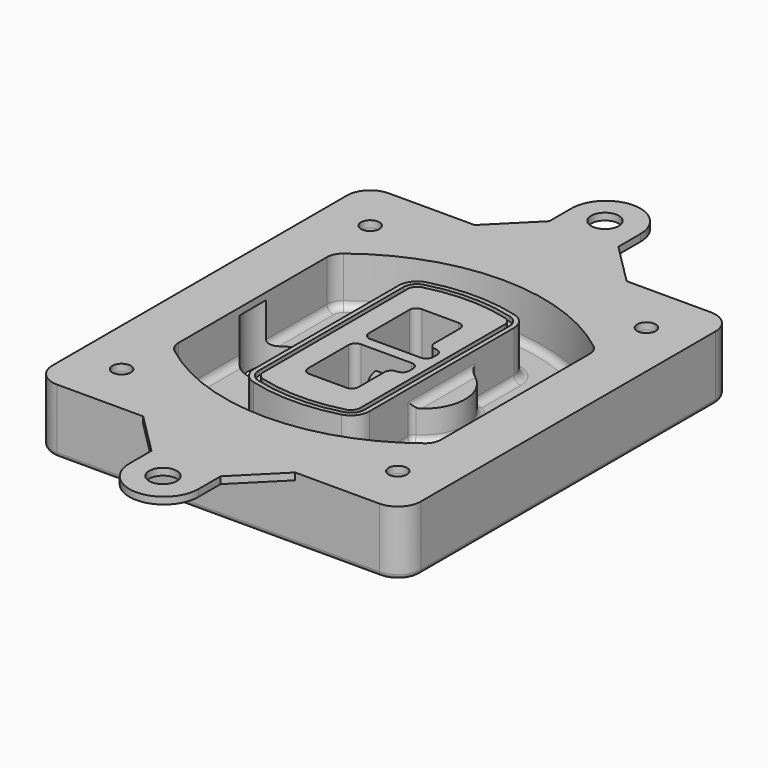
from build123d import *

# Parameters (mm, degrees)
F0_R      = 4
F1_DEPTH  = 25
F2_DEPTH  = 3
F3_DEPTH  = 18
F5_DEPTH  = 21
F6_DEPTH  = 2
F8_DEPTH  = 20
F9_DEPTH  = 16
F10_DEPTH = 25
F7_R      = 6
F7_R_2    = 4
F11_DEPTH = 6
F13_DEPTH = 9
F14_R     = 2
F15_R     = 3
F16_R     = 4
F16_R_2   = 6.0213144339
F17_DEPTH = 3


# Not quite as in the source:
# - a feature names something its author has since deleted; it is built from what else it names


with BuildPart() as f1:
    # F0 (on Top) → F1 (new body)
    with BuildSketch(Plane.XY):
        with BuildLine():
            ThreePointArc((-80, -80), (-77.0710678119, -87.0710678119), (-70, -90))
            Line((-70, -90), (70, -90))
            ThreePointArc((70, -90), (77.0710678119, -87.0710678119), (80, -80))
            Line((80, -80), (80, 80))
            ThreePointArc((80, 80), (77.0710678119, 87.0710678119), (70, 90))
            Line((70, 90), (-70, 90))
            ThreePointArc((-70, 90), (-77.0710678119, 87.0710678119), (-80, 80))
            Line((-80, 80), (-80, -80))
        make_face()
        with Locations((-60, -67.5)):
            Circle(F0_R, mode=Mode.SUBTRACT)
        with Locations((60, -67.5)):
            Circle(F0_R, mode=Mode.SUBTRACT)
        with Locations((-60, 67.5)):
            Circle(F0_R, mode=Mode.SUBTRACT)
        with BuildLine():
            ThreePointArc((-64, 40.2934422872), (-62.5820384798, 46.4328484224), (-58.6153846154, 51.3286200352))
            ThreePointArc((-58.6153846154, 51.3286200352), (0, 71.5), (58.6153846154, 51.3286200352))
            ThreePointArc((58.6153846154, 51.3286200352), (62.5820384798, 46.4328484224), (64, 40.2934422872))
            Line((64, 40.2934422872), (64, -40.2934422872))
            ThreePointArc((64, -40.2934422872), (62.5820384798, -46.4328484224), (58.6153846154, -51.3286200352))
            ThreePointArc((58.6153846154, -51.3286200352), (0, -71.5), (-58.6153846154, -51.3286200352))
            ThreePointArc((-58.6153846154, -51.3286200352), (-62.5820384798, -46.4328484224), (-64, -40.2934422872))
            Line((-64, -40.2934422872), (-64, 40.2934422872))
        make_face(mode=Mode.SUBTRACT)
        with Locations((60, 67.5)):
            Circle(F0_R, mode=Mode.SUBTRACT)
        with BuildLine():
            ThreePointArc((58.6153846154, 51.3286200352), (0, 71.5), (-58.6153846154, 51.3286200352))
            ThreePointArc((-58.6153846154, 51.3286200352), (-62.5820384798, 46.4328484224), (-64, 40.2934422872))
            Line((-64, 40.2934422872), (-64, -40.2934422872))
            ThreePointArc((-64, -40.2934422872), (-62.5820384798, -46.4328484224), (-58.6153846154, -51.3286200352))
            ThreePointArc((-58.6153846154, -51.3286200352), (0, -71.5), (58.6153846154, -51.3286200352))
            ThreePointArc((58.6153846154, -51.3286200352), (62.5820384798, -46.4328484224), (64, -40.2934422872))
            Line((64, -40.2934422872), (64, 40.2934422872))
            ThreePointArc((64, 40.2934422872), (62.5820384798, 46.4328484224), (58.6153846154, 51.3286200352))
        make_face()
        with BuildLine():
            Line((-60, -40.2934422872), (-60, 40.2934422872))
            ThreePointArc((-60, 40.2934422872), (-58.9871703427, 44.6787323838), (-56.1538461538, 48.1757121072))
            ThreePointArc((-56.1538461538, 48.1757121072), (0, 67.5), (56.1538461538, 48.1757121072))
            ThreePointArc((56.1538461538, 48.1757121072), (58.9871703427, 44.6787323838), (60, 40.2934422872))
            Line((60, 40.2934422872), (60, -40.2934422872))
            ThreePointArc((60, -40.2934422872), (58.9871703427, -44.6787323838), (56.1538461538, -48.1757121072))
            ThreePointArc((56.1538461538, -48.1757121072), (0, -67.5), (-56.1538461538, -48.1757121072))
            ThreePointArc((-56.1538461538, -48.1757121072), (-58.9871703427, -44.6787323838), (-60, -40.2934422872))
        make_face(mode=Mode.SUBTRACT)
        with BuildLine():
            ThreePointArc((-56.1538461538, 48.1757121072), (-58.9871703427, 44.6787323838), (-60, 40.2934422872))
            Line((-60, 40.2934422872), (-60, -40.2934422872))
            ThreePointArc((-60, -40.2934422872), (-58.9871703427, -44.6787323838), (-56.1538461538, -48.1757121072))
            ThreePointArc((-56.1538461538, -48.1757121072), (0, -67.5), (56.1538461538, -48.1757121072))
            ThreePointArc((56.1538461538, -48.1757121072), (58.9871703427, -44.6787323838), (60, -40.2934422872))
            Line((60, -40.2934422872), (60, 40.2934422872))
            ThreePointArc((60, 40.2934422872), (58.9871703427, 44.6787323838), (56.1538461538, 48.1757121072))
            ThreePointArc((56.1538461538, 48.1757121072), (0, 67.5), (-56.1538461538, 48.1757121072))
        make_face()
        with BuildLine():
            ThreePointArc((54.3076923077, 45.8110311612), (56.2910192399, 43.3631453548), (57, 40.2934422872))
            Line((57, 40.2934422872), (57, -40.2934422872))
            ThreePointArc((57, -40.2934422872), (56.2910192399, -43.3631453548), (54.3076923077, -45.8110311612))
            ThreePointArc((54.3076923077, -45.8110311612), (0, -64.5), (-54.3076923077, -45.8110311612))
            ThreePointArc((-54.3076923077, -45.8110311612), (-56.2910192399, -43.3631453548), (-57, -40.2934422872))
            Line((-57, -40.2934422872), (-57, 40.2934422872))
            ThreePointArc((-57, 40.2934422872), (-56.2910192399, 43.3631453548), (-54.3076923077, 45.8110311612))
            ThreePointArc((-54.3076923077, 45.8110311612), (0, 64.5), (54.3076923077, 45.8110311612))
        make_face(mode=Mode.SUBTRACT)
        with BuildLine():
            Line((57, -40.2934422872), (57, 40.2934422872))
            ThreePointArc((57, 40.2934422872), (56.2910192399, 43.3631453548), (54.3076923077, 45.8110311612))
            ThreePointArc((54.3076923077, 45.8110311612), (0, 64.5), (-54.3076923077, 45.8110311612))
            ThreePointArc((-54.3076923077, 45.8110311612), (-56.2910192399, 43.3631453548), (-57, 40.2934422872))
            Line((-57, 40.2934422872), (-57, -40.2934422872))
            ThreePointArc((-57, -40.2934422872), (-56.2910192399, -43.3631453548), (-54.3076923077, -45.8110311612))
            ThreePointArc((-54.3076923077, -45.8110311612), (0, -64.5), (54.3076923077, -45.8110311612))
            ThreePointArc((54.3076923077, -45.8110311612), (56.2910192399, -43.3631453548), (57, -40.2934422872))
        make_face()
    extrude(amount=-F1_DEPTH)

    # F0 (on Top) → F2 (join)
    with BuildSketch(Plane.XY):
        with BuildLine():
            ThreePointArc((-56.1538461538, 48.1757121072), (-58.9871703427, 44.6787323838), (-60, 40.2934422872))
            Line((-60, 40.2934422872), (-60, -40.2934422872))
            ThreePointArc((-60, -40.2934422872), (-58.9871703427, -44.6787323838), (-56.1538461538, -48.1757121072))
            ThreePointArc((-56.1538461538, -48.1757121072), (0, -67.5), (56.1538461538, -48.1757121072))
            ThreePointArc((56.1538461538, -48.1757121072), (58.9871703427, -44.6787323838), (60, -40.2934422872))
            Line((60, -40.2934422872), (60, 40.2934422872))
            ThreePointArc((60, 40.2934422872), (58.9871703427, 44.6787323838), (56.1538461538, 48.1757121072))
            ThreePointArc((56.1538461538, 48.1757121072), (0, 67.5), (-56.1538461538, 48.1757121072))
        make_face()
        with BuildLine():
            ThreePointArc((54.3076923077, 45.8110311612), (56.2910192399, 43.3631453548), (57, 40.2934422872))
            Line((57, 40.2934422872), (57, -40.2934422872))
            ThreePointArc((57, -40.2934422872), (56.2910192399, -43.3631453548), (54.3076923077, -45.8110311612))
            ThreePointArc((54.3076923077, -45.8110311612), (0, -64.5), (-54.3076923077, -45.8110311612))
            ThreePointArc((-54.3076923077, -45.8110311612), (-56.2910192399, -43.3631453548), (-57, -40.2934422872))
            Line((-57, -40.2934422872), (-57, 40.2934422872))
            ThreePointArc((-57, 40.2934422872), (-56.2910192399, 43.3631453548), (-54.3076923077, 45.8110311612))
            ThreePointArc((-54.3076923077, 45.8110311612), (0, 64.5), (54.3076923077, 45.8110311612))
        make_face(mode=Mode.SUBTRACT)
    extrude(amount=F2_DEPTH)

    # F0 (on Top) → F3 (cut)
    with BuildSketch(Plane.XY):
        with BuildLine():
            Line((57, -40.2934422872), (57, 40.2934422872))
            ThreePointArc((57, 40.2934422872), (56.2910192399, 43.3631453548), (54.3076923077, 45.8110311612))
            ThreePointArc((54.3076923077, 45.8110311612), (0, 64.5), (-54.3076923077, 45.8110311612))
            ThreePointArc((-54.3076923077, 45.8110311612), (-56.2910192399, 43.3631453548), (-57, 40.2934422872))
            Line((-57, 40.2934422872), (-57, -40.2934422872))
            ThreePointArc((-57, -40.2934422872), (-56.2910192399, -43.3631453548), (-54.3076923077, -45.8110311612))
            ThreePointArc((-54.3076923077, -45.8110311612), (0, -64.5), (54.3076923077, -45.8110311612))
            ThreePointArc((54.3076923077, -45.8110311612), (56.2910192399, -43.3631453548), (57, -40.2934422872))
        make_face()
    extrude(amount=-F3_DEPTH, mode=Mode.SUBTRACT)

    # F4 (on face) → F5 (join, through all)
    with BuildSketch(Plane.XY.offset(3)):
        with BuildLine():
            ThreePointArc((-25, -39.2465276821), (-23.3511545998, -44.1109737193), (-19.0842911877, -46.9702398883))
            ThreePointArc((-19.0842911877, -46.9702398883), (0, -49.5), (19.0842911877, -46.9702398883))
            ThreePointArc((19.0842911877, -46.9702398883), (23.3511545998, -44.1109737193), (25, -39.2465276821))
            Line((25, -39.2465276821), (25, 39.2465276821))
            ThreePointArc((25, 39.2465276821), (23.3511545998, 44.1109737193), (19.0842911877, 46.9702398883))
            ThreePointArc((19.0842911877, 46.9702398883), (0, 49.5), (-19.0842911877, 46.9702398883))
            ThreePointArc((-19.0842911877, 46.9702398883), (-23.3511545998, 44.1109737193), (-25, 39.2465276821))
            Line((-25, 39.2465276821), (-25, -39.2465276821))
        make_face()
        with BuildLine():
            ThreePointArc((18.5632183908, 45.0393118368), (21.7633659499, 42.89486221), (23, 39.2465276821))
            Line((23, 39.2465276821), (23, -39.2465276821))
            ThreePointArc((23, -39.2465276821), (21.7633659499, -42.89486221), (18.5632183908, -45.0393118368))
            ThreePointArc((18.5632183908, -45.0393118368), (0, -47.5), (-18.5632183908, -45.0393118368))
            ThreePointArc((-18.5632183908, -45.0393118368), (-21.7633659499, -42.89486221), (-23, -39.2465276821))
            Line((-23, -39.2465276821), (-23, 39.2465276821))
            ThreePointArc((-23, 39.2465276821), (-21.7633659499, 42.89486221), (-18.5632183908, 45.0393118368))
            ThreePointArc((-18.5632183908, 45.0393118368), (0, 47.5), (18.5632183908, 45.0393118368))
        make_face(mode=Mode.SUBTRACT)
        with BuildLine():
            Line((23, -39.2465276821), (23, 39.2465276821))
            ThreePointArc((23, 39.2465276821), (21.7633659499, 42.89486221), (18.5632183908, 45.0393118368))
            ThreePointArc((18.5632183908, 45.0393118368), (0, 47.5), (-18.5632183908, 45.0393118368))
            ThreePointArc((-18.5632183908, 45.0393118368), (-21.7633659499, 42.89486221), (-23, 39.2465276821))
            Line((-23, 39.2465276821), (-23, -39.2465276821))
            ThreePointArc((-23, -39.2465276821), (-21.7633659499, -42.89486221), (-18.5632183908, -45.0393118368))
            ThreePointArc((-18.5632183908, -45.0393118368), (0, -47.5), (18.5632183908, -45.0393118368))
            ThreePointArc((18.5632183908, -45.0393118368), (21.7633659499, -42.89486221), (23, -39.2465276821))
        make_face()
        with BuildLine():
            ThreePointArc((18.0421455939, 43.1083837852), (20.1755772999, 41.6787507007), (21, 39.2465276821))
            Line((21, 39.2465276821), (21, -39.2465276821))
            ThreePointArc((21, -39.2465276821), (20.1755772999, -41.6787507007), (18.0421455939, -43.1083837852))
            ThreePointArc((18.0421455939, -43.1083837852), (0, -45.5), (-18.0421455939, -43.1083837852))
            ThreePointArc((-18.0421455939, -43.1083837852), (-20.1755772999, -41.6787507007), (-21, -39.2465276821))
            Line((-21, -39.2465276821), (-21, 39.2465276821))
            ThreePointArc((-21, 39.2465276821), (-20.1755772999, 41.6787507007), (-18.0421455939, 43.1083837852))
            ThreePointArc((-18.0421455939, 43.1083837852), (0, 45.5), (18.0421455939, 43.1083837852))
        make_face(mode=Mode.SUBTRACT)
        with BuildLine():
            Line((21, -39.2465276821), (21, 39.2465276821))
            ThreePointArc((21, 39.2465276821), (20.1755772999, 41.6787507007), (18.0421455939, 43.1083837852))
            ThreePointArc((18.0421455939, 43.1083837852), (0, 45.5), (-18.0421455939, 43.1083837852))
            ThreePointArc((-18.0421455939, 43.1083837852), (-20.1755772999, 41.6787507007), (-21, 39.2465276821))
            Line((-21, 39.2465276821), (-21, -39.2465276821))
            ThreePointArc((-21, -39.2465276821), (-20.1755772999, -41.6787507007), (-18.0421455939, -43.1083837852))
            ThreePointArc((-18.0421455939, -43.1083837852), (0, -45.5), (18.0421455939, -43.1083837852))
            ThreePointArc((18.0421455939, -43.1083837852), (20.1755772999, -41.6787507007), (21, -39.2465276821))
        make_face()
        with BuildLine():
            Line((-8, -2.5), (14, -2.5))
            ThreePointArc((14, -2.5), (16.1213203436, -3.3786796564), (17, -5.5))
            Line((17, -5.5), (17, -7.5))
            ThreePointArc((17, -7.5), (16.1213203436, -9.6213203436), (14, -10.5))
            ThreePointArc((14, -10.5), (11.8786796564, -11.3786796564), (11, -13.5))
            Line((11, -13.5), (11, -27.5))
            ThreePointArc((11, -27.5), (10.1213203436, -29.6213203436), (8, -30.5))
            Line((8, -30.5), (-8, -30.5))
            ThreePointArc((-8, -30.5), (-10.1213203436, -29.6213203436), (-11, -27.5))
            Line((-11, -27.5), (-11, -5.5))
            ThreePointArc((-11, -5.5), (-10.1213203436, -3.3786796564), (-8, -2.5))
        make_face(mode=Mode.SUBTRACT)
        with BuildLine():
            ThreePointArc((-8, 2.5), (-10.1213203436, 3.3786796564), (-11, 5.5))
            Line((-11, 5.5), (-11, 27.5))
            ThreePointArc((-11, 27.5), (-10.1213203436, 29.6213203436), (-8, 30.5))
            Line((-8, 30.5), (8, 30.5))
            ThreePointArc((8, 30.5), (10.1213203436, 29.6213203436), (11, 27.5))
            Line((11, 27.5), (11, 13.5))
            ThreePointArc((11, 13.5), (11.8786796564, 11.3786796564), (14, 10.5))
            ThreePointArc((14, 10.5), (16.1213203436, 9.6213203436), (17, 7.5))
            Line((17, 7.5), (17, 5.5))
            ThreePointArc((17, 5.5), (16.1213203436, 3.3786796564), (14, 2.5))
            Line((14, 2.5), (-8, 2.5))
        make_face(mode=Mode.SUBTRACT)
    extrude(amount=-F5_DEPTH)

    # F4 (on face) → F6 (cut)
    with BuildSketch(Plane.XY.offset(3)):
        with BuildLine():
            Line((23, -39.2465276821), (23, 39.2465276821))
            ThreePointArc((23, 39.2465276821), (21.7633659499, 42.89486221), (18.5632183908, 45.0393118368))
            ThreePointArc((18.5632183908, 45.0393118368), (0, 47.5), (-18.5632183908, 45.0393118368))
            ThreePointArc((-18.5632183908, 45.0393118368), (-21.7633659499, 42.89486221), (-23, 39.2465276821))
            Line((-23, 39.2465276821), (-23, -39.2465276821))
            ThreePointArc((-23, -39.2465276821), (-21.7633659499, -42.89486221), (-18.5632183908, -45.0393118368))
            ThreePointArc((-18.5632183908, -45.0393118368), (0, -47.5), (18.5632183908, -45.0393118368))
            ThreePointArc((18.5632183908, -45.0393118368), (21.7633659499, -42.89486221), (23, -39.2465276821))
        make_face()
        with BuildLine():
            ThreePointArc((18.0421455939, 43.1083837852), (20.1755772999, 41.6787507007), (21, 39.2465276821))
            Line((21, 39.2465276821), (21, -39.2465276821))
            ThreePointArc((21, -39.2465276821), (20.1755772999, -41.6787507007), (18.0421455939, -43.1083837852))
            ThreePointArc((18.0421455939, -43.1083837852), (0, -45.5), (-18.0421455939, -43.1083837852))
            ThreePointArc((-18.0421455939, -43.1083837852), (-20.1755772999, -41.6787507007), (-21, -39.2465276821))
            Line((-21, -39.2465276821), (-21, 39.2465276821))
            ThreePointArc((-21, 39.2465276821), (-20.1755772999, 41.6787507007), (-18.0421455939, 43.1083837852))
            ThreePointArc((-18.0421455939, 43.1083837852), (0, 45.5), (18.0421455939, 43.1083837852))
        make_face(mode=Mode.SUBTRACT)
    extrude(amount=-F6_DEPTH, mode=Mode.SUBTRACT)

    # F7 (on face) → F8 (join)
    with BuildSketch(Plane(origin=(0, 0, -25), x_dir=(1, 0, 0), z_dir=(0, 0, -1))):
        with BuildLine():
            ThreePointArc((3.28842436, 0), (16.7567035675, 13.4682792075), (30.224982775, 0))
            Line((30.224982775, 0), (35.224982775, 0))
            ThreePointArc((35.224982775, 0), (16.7567035675, 18.4682792075), (-1.71157564, 0))
            Line((-1.71157564, 0), (3.28842436, 0))
        make_face()
        with BuildLine():
            Line((3.28842436, 0), (30.224982775, 0))
            ThreePointArc((30.224982775, 0), (16.7567035675, 13.4682792075), (3.28842436, 0))
        make_face()
        with BuildLine():
            ThreePointArc((3.28842436, 0), (16.7567035675, -13.4682792075), (30.224982775, 0))
            Line((30.224982775, 0), (3.28842436, 0))
        make_face()
        with BuildLine():
            Line((35.224982775, 0), (30.224982775, 0))
            ThreePointArc((30.224982775, 0), (16.7567035675, -13.4682792075), (3.28842436, 0))
            Line((3.28842436, 0), (-1.71157564, 0))
            ThreePointArc((-1.71157564, 0), (16.7567035675, -18.4682792075), (35.224982775, 0))
        make_face()
    extrude(amount=-F8_DEPTH)

    # F7 (on face) → F9 (cut)
    with BuildSketch(Plane(origin=(0, 0, -25), x_dir=(1, 0, 0), z_dir=(0, 0, -1))):
        with BuildLine():
            Line((3.28842436, 0), (30.224982775, 0))
            ThreePointArc((30.224982775, 0), (16.7567035675, 13.4682792075), (3.28842436, 0))
        make_face()
        with BuildLine():
            ThreePointArc((3.28842436, 0), (16.7567035675, -13.4682792075), (30.224982775, 0))
            Line((30.224982775, 0), (3.28842436, 0))
        make_face()
    extrude(amount=-F9_DEPTH, mode=Mode.SUBTRACT)

    # F7 (on face) → F10 (cut)
    with BuildSketch(Plane(origin=(0, 0, -25), x_dir=(1, 0, 0), z_dir=(0, 0, -1))):
        with BuildLine():
            Line((-59.0318229325, 0), (-32.0952645175, 0))
            ThreePointArc((-32.0952645175, 0), (-45.563543725, 13.4682792075), (-59.0318229325, 0))
        make_face()
        with BuildLine():
            ThreePointArc((-59.0318229325, 0), (-45.563543725, -13.4682792075), (-32.0952645175, 0))
            Line((-32.0952645175, 0), (-59.0318229325, 0))
        make_face()
    extrude(amount=-F10_DEPTH, mode=Mode.SUBTRACT)

    # F7 (on face) → F11 (cut)
    with BuildSketch(Plane(origin=(0, 0, -25), x_dir=(1, 0, 0), z_dir=(0, 0, -1))):
        with Locations((60, -67.5)):
            Circle(F7_R)
        with Locations((60, -67.5)):
            Circle(F7_R_2, mode=Mode.SUBTRACT)
        with Locations((-60, -67.5)):
            Circle(F7_R)
        with Locations((-60, -67.5)):
            Circle(F7_R_2, mode=Mode.SUBTRACT)
        with Locations((-60, 67.5)):
            Circle(F7_R)
        with Locations((-60, 67.5)):
            Circle(F7_R_2, mode=Mode.SUBTRACT)
        with Locations((60, 67.5)):
            Circle(F7_R)
        with Locations((60, 67.5)):
            Circle(F7_R_2, mode=Mode.SUBTRACT)
    extrude(amount=-F11_DEPTH, mode=Mode.SUBTRACT)

    # F12 (on face) → F13 (cut, through all)
    with BuildSketch(Plane(origin=(0, 0, -9), x_dir=(1, 0, 0), z_dir=(0, 0, -1))):
        with BuildLine():
            Line((11, 13.5), (11, 17.5481537753))
            ThreePointArc((11, 17.5481537753), (2.5696536419, 11.8239143813), (-1.5415842455, 2.5))
            Line((-1.5415842455, 2.5), (3.5224848595, 2.5))
            ThreePointArc((3.5224848595, 2.5), (6.1857188154, 8.3455872281), (11.2536447004, 12.2927168648))
            ThreePointArc((11.2536447004, 12.2927168648), (11.0640958889, 12.8831798879), (11, 13.5))
        make_face()
        with BuildLine():
            ThreePointArc((11.2536447004, -12.2927168648), (6.1857188154, -8.3455872281), (3.5224848595, -2.5))
            Line((3.5224848595, -2.5), (-1.5415842455, -2.5))
            ThreePointArc((-1.5415842455, -2.5), (2.5696536419, -11.8239143813), (11, -17.5481537753))
            Line((11, -17.5481537753), (11, -13.5))
            ThreePointArc((11, -13.5), (11.0640958889, -12.8831798879), (11.2536447004, -12.2927168648))
        make_face()
        with BuildLine():
            ThreePointArc((11.2536447004, 12.2927168648), (6.1857188154, 8.3455872281), (3.5224848595, 2.5))
            Line((3.5224848595, 2.5), (14, 2.5))
            ThreePointArc((14, 2.5), (16.1213203436, 3.3786796564), (17, 5.5))
            Line((17, 5.5), (17, 7.5))
            ThreePointArc((17, 7.5), (16.1213203436, 9.6213203436), (14, 10.5))
            ThreePointArc((14, 10.5), (12.3601599782, 10.9878446101), (11.2536447004, 12.2927168648))
        make_face()
        with BuildLine():
            Line((14, -2.5), (3.5224848595, -2.5))
            ThreePointArc((3.5224848595, -2.5), (6.1857188154, -8.3455872281), (11.2536447004, -12.2927168648))
            ThreePointArc((11.2536447004, -12.2927168648), (12.3601599782, -10.9878446101), (14, -10.5))
            ThreePointArc((14, -10.5), (16.1213203436, -9.6213203436), (17, -7.5))
            Line((17, -7.5), (17, -5.5))
            ThreePointArc((17, -5.5), (16.1213203436, -3.3786796564), (14, -2.5))
        make_face()
    extrude(amount=F13_DEPTH, mode=Mode.SUBTRACT)

    # F14
    f14_edges = [f1.edges().sort_by_distance(p)[0] for p in [
        (0, -90, -25),
    ]]
    fillet(f14_edges, radius=F14_R)

    # F15
    f15_edges = [f1.edges().sort_by_distance(p)[0] for p in [
        (-57, -23.703476, -18),
        (-57, 23.703476, -18),
        (25, 0, -5),
        (25, 16.526506, -11.5),
        (25, -16.526506, -11.5),
        (25, -27.886517, -18),
        (35.224983, 0, -18),
    ]]
    fillet(f15_edges, radius=F15_R)

    # F16 (on face) → F17 (join, through all)
    with BuildSketch(Plane.XY):
        with BuildLine():
            Line((33.3890186287, 90), (-32.6099851301, 90))
            Line((-32.6099851301, 90), (-70, 90))
            ThreePointArc((-70, 90), (-77.0710678119, 87.0710678119), (-80, 80))
            Line((-80, 80), (-80, -80))
            ThreePointArc((-80, -80), (-77.0710678119, -87.0710678119), (-70, -90))
            Line((-70, -90), (-32.6099851301, -90))
            Line((-32.6099851301, -90), (33.3890186287, -90))
            Line((33.3890186287, -90), (70, -90))
            ThreePointArc((70, -90), (77.0710678119, -87.0710678119), (80, -80))
            Line((80, -80), (80, 80))
            ThreePointArc((80, 80), (77.0710678119, 87.0710678119), (70, 90))
            Line((70, 90), (33.3890186287, 90))
        make_face()
        with Locations((-60, -67.5)):
            Circle(F16_R, mode=Mode.SUBTRACT)
        with Locations((60, -67.5)):
            Circle(F16_R, mode=Mode.SUBTRACT)
        with Locations((-60, 67.5)):
            Circle(F16_R, mode=Mode.SUBTRACT)
        with BuildLine():
            ThreePointArc((-60, 40.2934422872), (-58.9871703427, 44.6787323838), (-56.1538461538, 48.1757121072))
            ThreePointArc((-56.1538461538, 48.1757121072), (0, 67.5), (56.1538461538, 48.1757121072))
            ThreePointArc((56.1538461538, 48.1757121072), (58.9871703427, 44.6787323838), (60, 40.2934422872))
            Line((60, 40.2934422872), (60, -40.2934422872))
            ThreePointArc((60, -40.2934422872), (58.9871703427, -44.6787323838), (56.1538461538, -48.1757121072))
            ThreePointArc((56.1538461538, -48.1757121072), (0, -67.5), (-56.1538461538, -48.1757121072))
            ThreePointArc((-56.1538461538, -48.1757121072), (-58.9871703427, -44.6787323838), (-60, -40.2934422872))
            Line((-60, -40.2934422872), (-60, 40.2934422872))
        make_face(mode=Mode.SUBTRACT)
        with Locations((60, 67.5)):
            Circle(F16_R, mode=Mode.SUBTRACT)
        with BuildLine():
            Line((-14.6099851301, 108), (-32.6099851301, 90))
            Line((-32.6099851301, 90), (33.3890186287, 90))
            Line((33.3890186287, 90), (15.3890186287, 108))
            Line((15.3890186287, 108), (15.3890186287, 120))
            ThreePointArc((15.3890186287, 120), (0.3025790005, 134.9997509376), (-14.6099851301, 119.8271236141))
            Line((-14.6099851301, 119.8271236141), (-14.6099851301, 108))
        make_face()
        with Locations((0, 120)):
            Circle(F16_R_2, mode=Mode.SUBTRACT)
        with BuildLine():
            Line((33.3890186287, -90), (-32.6099851301, -90))
            Line((-32.6099851301, -90), (-14.6099851301, -108))
            Line((-14.6099851301, -108), (-14.6099851301, -119.8271236141))
            ThreePointArc((-14.6099851301, -119.8271236141), (0.3025790005, -134.9997509376), (15.3890186287, -120))
            Line((15.3890186287, -120), (15.3890186287, -108))
            Line((15.3890186287, -108), (33.3890186287, -90))
        make_face()
        with Locations((0, -120)):
            Circle(F16_R_2, mode=Mode.SUBTRACT)
    extrude(amount=F17_DEPTH)


solid = f1.part
